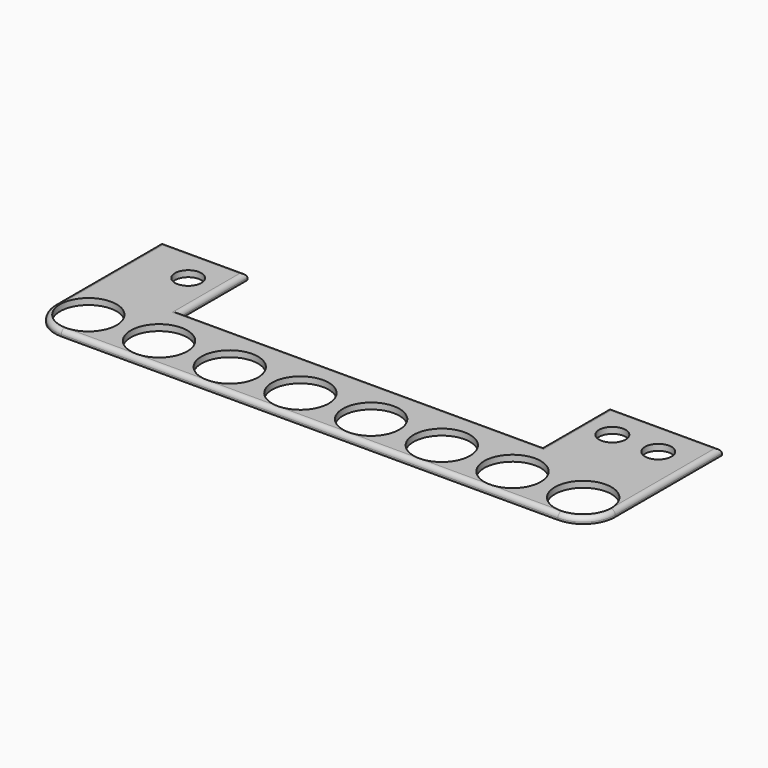
from build123d import *

# Parameters (mm, degrees)
F0_R        = 3.2
F0_R_2      = 1.5
F1_DEPTH    = 0.7
F2_R        = 0.49999
F3_T1_DEPTH = 9.7
F3_T4_ANGLE = 90
F3_T6_ANGLE = 90


# Not quite as in the source:
# - a fillet or chamfer that OpenCascade refuses, or shapes differently, is made with other operations: its cross-section is extruded or revolved along the edge and cut away or added
# - a fillet or chamfer is up to 0.001 mm smaller than in the source, because OpenCascade refuses the exact size
# - a feature names something its author has since deleted; it is built from what else it names


with BuildPart() as f1:
    # F0 (on Top) → F1 (new body)
    with BuildSketch(Plane.XY):
        Polygon((-22, 18.7), (-31.7, 18.7), (-31.7, 0), (-18.3513443917, 0), (-10.3513443917, 0), (31.7, 0), (31.7, 18.7), (19, 18.7), (19, 9.2), (-22, 9.2), align=None)
        with Locations((-28, 3.7)):
            Circle(F0_R, mode=Mode.SUBTRACT)
        with Locations((-20, 3.7)):
            Circle(F0_R, mode=Mode.SUBTRACT)
        with Locations((-12, 3.7)):
            Circle(F0_R, mode=Mode.SUBTRACT)
        with Locations((-4, 3.7)):
            Circle(F0_R, mode=Mode.SUBTRACT)
        with Locations((4, 3.7)):
            Circle(F0_R, mode=Mode.SUBTRACT)
        with Locations((12, 3.7)):
            Circle(F0_R, mode=Mode.SUBTRACT)
        with Locations((20, 3.7)):
            Circle(F0_R, mode=Mode.SUBTRACT)
        with Locations((28, 3.7)):
            Circle(F0_R, mode=Mode.SUBTRACT)
        with Locations((-25.5, 14.7)):
            Circle(F0_R_2, mode=Mode.SUBTRACT)
        with Locations((22.5, 14.7)):
            Circle(F0_R_2, mode=Mode.SUBTRACT)
        with Locations((27.7, 14.7)):
            Circle(F0_R_2, mode=Mode.SUBTRACT)
    extrude(amount=F1_DEPTH)

    # F2 (radius 0.5 in the source; OpenCascade refuses exactly that, so slightly less here)
    f2_edges = [f1.edges().sort_by_distance(p)[0] for p in [
        (0, 0, 0.7),
        (-31.7, 9.35, 0.7),
        (-26.85, 18.7, 0.7),
        (-22, 13.95, 0.7),
        (-1.5, 9.2, 0.7),
        (19, 13.95, 0.7),
        (25.35, 18.7, 0.7),
        (31.7, 9.35, 0.7),
    ]]
    fillet(f2_edges, radius=F2_R)

    # F3: fillet of radius 3.6 on 4 edges, made by hand

    # F3_s2 → F3_t1 (cut)
    with BuildSketch(Plane.XY.offset(-9)):
        with BuildLine():
            ThreePointArc((-28.1, 0), (-30.6455844123, 1.0544155877), (-31.7, 3.6))
            Line((-31.7, 3.6), (-31.7, 0))
            Line((-31.7, 0), (-28.1, 0))
        make_face()
        with BuildLine():
            ThreePointArc((28.1, 0), (30.6455844123, 1.0544155877), (31.7, 3.6))
            Line((31.7, 3.6), (31.7, 0))
            Line((31.7, 0), (28.1, 0))
        make_face()
    extrude(amount=F3_T1_DEPTH, mode=Mode.SUBTRACT)

    # F3_s3 → F3_t4 (revolve, cut)
    with BuildSketch(Plane.XZ.offset(-3.6)):
        with BuildLine():
            ThreePointArc((-31.20001, 0.7), (-31.5535563195, 0.5535563195), (-31.7, 0.20001))
            Line((-31.7, 0.20001), (-31.7, 0.7))
            Line((-31.7, 0.7), (-31.20001, 0.7))
        make_face()
    revolve(axis=Axis((-28.1, 3.6, 0.7), (0, 0, 1)), revolution_arc=F3_T4_ANGLE, mode=Mode.SUBTRACT)

    # F3_s5 → F3_t6 (revolve, cut)
    with BuildSketch(Plane.YZ.offset(28.1)):
        with BuildLine():
            ThreePointArc((0.49999, 0.7), (0.1464436805, 0.5535563195), (0, 0.20001))
            Line((0, 0.20001), (0, 0.7))
            Line((0, 0.7), (0.49999, 0.7))
        make_face()
    revolve(axis=Axis((28.1, 3.6, 0.7), (0, 0, 1)), revolution_arc=F3_T6_ANGLE, mode=Mode.SUBTRACT)


solid = f1.part
